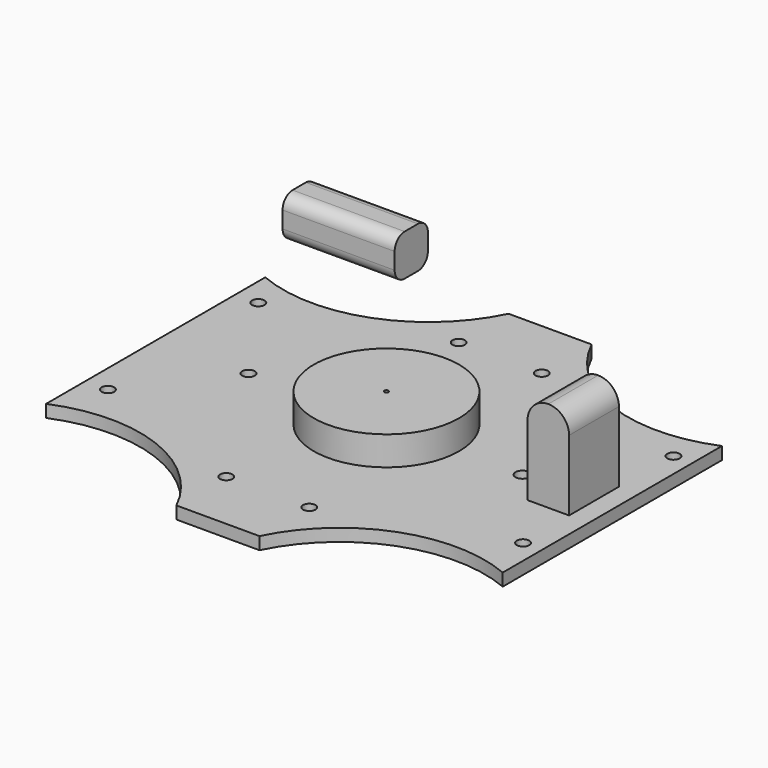
from build123d import *

# Parameters (mm, degrees)
F0_R     = 17.5
F0_R_2   = 0.5
F1_DEPTH = 10
F2_W     = 27
F2_H     = 10
F3_DEPTH = 10
F4_R     = 3
F5_R     = 1.5
F5_R_2   = 1.7887858733
F5_R_3   = 1.6766314054
F6_DEPTH = 3
F7_W     = 10
F7_H     = 15
F8_DEPTH = 25
F9_R     = 4.99999


# Not quite as in the source:
# - a fillet or chamfer is up to 0.001 mm smaller than in the source, because OpenCascade refuses the exact size


with BuildPart() as f1:
    # F0 (on Top) → F1 (new body)
    with BuildSketch(Plane.XY):
        Circle(F0_R)
        Circle(F0_R_2, mode=Mode.SUBTRACT)
    extrude(amount=F1_DEPTH)


with BuildPart() as f3:
    # F2 (on Top) → F3 (new body)
    with BuildSketch(Plane.XY):
        with Locations((-51.5112442672, 54.997754395)):
            Rectangle(F2_W, F2_H)
    extrude(amount=F3_DEPTH)

    # F4
    f4_edges = [f3.edges().sort_by_distance(p)[0] for p in [
        (-51.511244, 59.997754, 10),
        (-51.511244, 49.997754, 10),
        (-51.511244, 49.997754, 0),
        (-51.511244, 59.997754, 0),
    ]]
    fillet(f4_edges, radius=F4_R)


with BuildPart() as f6:
    # F5 (on Top) → F6 (new body)
    with BuildSketch(Plane.XY):
        with BuildLine():
            ThreePointArc((54.7724512979, 32.5553555772), (28.8891229863, 32.099486517), (9.7724512979, 49.5553555772))
            Line((9.7724512979, 49.5553555772), (-10.2275487021, 49.5553555772))
            ThreePointArc((-10.2275487021, 49.5553555772), (-29.3442203904, 32.099486517), (-55.2275487021, 32.5553555772))
            Line((-55.2275487021, 32.5553555772), (-55.2275487021, -33.4446444228))
            ThreePointArc((-55.2275487021, -33.4446444228), (-29.3442203904, -32.9887753626), (-10.2275487021, -50.4446444228))
            Line((-10.2275487021, -50.4446444228), (9.7724512979, -50.4446444228))
            ThreePointArc((9.7724512979, -50.4446444228), (28.8891229863, -32.9887753626), (54.7724512979, -33.4446444228))
            Line((54.7724512979, -33.4446444228), (54.7724512979, 32.5553555772))
        make_face()
        with Locations((-10.2275487021, -35.4446444228)):
            Circle(F5_R, mode=Mode.SUBTRACT)
        with Locations((-49.7831985605, -21.6310646678)):
            Circle(F5_R, mode=Mode.SUBTRACT)
        with Locations((9.7724512979, -35.4446444228)):
            Circle(F5_R, mode=Mode.SUBTRACT)
        with Locations((50.2168014395, -21.6310646678)):
            Circle(F5_R, mode=Mode.SUBTRACT)
        with Locations((-33.2275487021, 0)):
            Circle(F5_R, mode=Mode.SUBTRACT)
        with Locations((-49.7831985605, 23.6533302814)):
            Circle(F5_R, mode=Mode.SUBTRACT)
        with Locations((-13.2275487021, 0)):
            Circle(F5_R_2, mode=Mode.SUBTRACT)
        with Locations((-10.2275487021, 34.5553555772)):
            Circle(F5_R, mode=Mode.SUBTRACT)
        with Locations((12.7724512979, 0)):
            Circle(F5_R, mode=Mode.SUBTRACT)
        with Locations((32.7724512979, 0)):
            Circle(F5_R_3, mode=Mode.SUBTRACT)
        with Locations((50.2168014395, 23.6533302814)):
            Circle(F5_R, mode=Mode.SUBTRACT)
        with Locations((9.7724512979, 34.5553555772)):
            Circle(F5_R, mode=Mode.SUBTRACT)
    extrude(amount=F6_DEPTH)

    # F7 (on Top) → F8 (join)
    with BuildSketch(Plane.XY):
        with Locations((45, 0)):
            Rectangle(F7_W, F7_H)
    extrude(amount=F8_DEPTH)

    # F9 (radius 5 in the source; OpenCascade refuses exactly that, so slightly less here)
    f9_edges = [f6.edges().sort_by_distance(p)[0] for p in [
        (50, 0, 25),
        (40, 0, 25),
    ]]
    fillet(f9_edges, radius=F9_R)


solid = Compound([f1.part, f3.part, f6.part])
